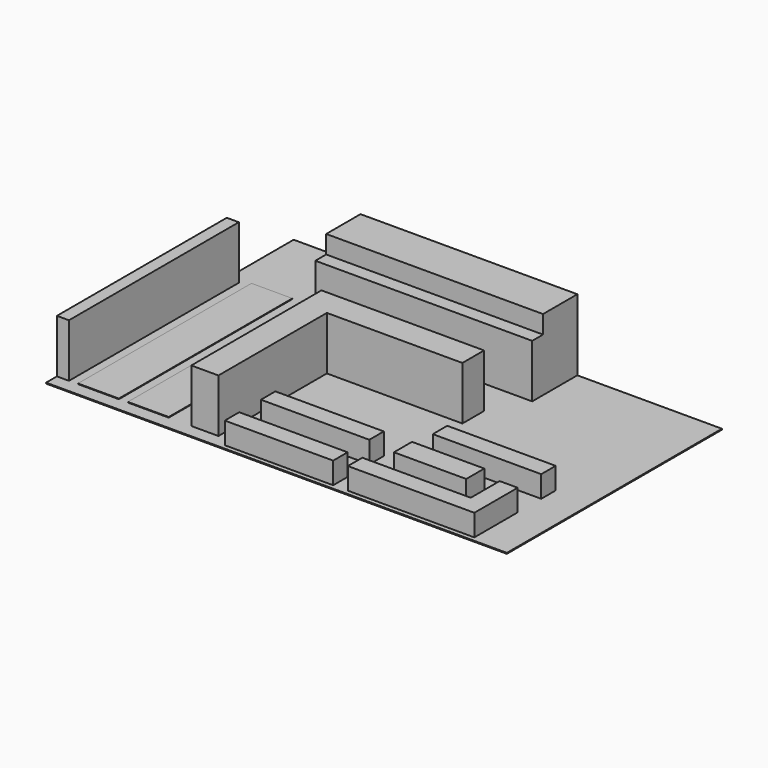
from build123d import *

# Parameters (mm, degrees)
F0_W     = 1377.95
F0_H     = 5486.4
F0_H_2   = 7315.2
F0_W_2   = 2438.4
F0_H_3   = 762
F0_W_3   = 3352.8
F0_H_4   = 1371.6
F0_W_4   = 914.4
F0_H_5   = 2438.4
F1_DEPTH = 30.48
F0_W_5   = 406.4
F0_H_6   = 7162.8
F0_W_6   = 7315.2
F0_H_7   = 457.2
F2_DEPTH = 1828.8
F0_W_7   = 1828.8
F0_H_8   = 609.6
F3_DEPTH = 762
F0_H_9   = 1447.8
F4_DEPTH = 2438.4
F6_DEPTH = 50.8
F0_W_8   = 457.2
F0_W_9   = 4572
F0_H_10  = 914.4
F7_DEPTH = 1828.8


# Not quite as in the source:
# - the program builds the solid bodies; features that only make, move or delete a surface that nothing else refers to are left out


with BuildPart() as f1:
    # F0 (on Top) → F1 (new body)
    with BuildSketch(Plane.XY):
        Polygon((3352.8, 9067.8), (0, 9067.8), (0, 7620), (406.4, 7620), (406.4, 457.2), (0, 457.2), (0, 0), (914.4, 0), (2438.4, 0), (5486.4, 0), (7010.4, 0), (13106.4, 0), (14630.4, 0), (14630.4, 2438.4), (15544.8, 2438.4), (15544.8, 3886.2), (10668, 3886.2), (10668, 7162.8), (3352.8, 7162.8), (3352.8, 7620), align=None)
        Polygon((5905.5, 1676.4), (5905.5, 2286), (7734.3, 2286), (9563.1, 2286), (9563.1, 1676.4), (9563.1, 762), (9563.1, 152.4), (7734.3, 152.4), (5905.5, 152.4), (5905.5, 762), align=None, mode=Mode.SUBTRACT)
        with Locations((3082.925, 3200.4)):
            Rectangle(F0_W, F0_H, mode=Mode.SUBTRACT)
        with Locations((1400.175, 4114.8)):
            Rectangle(F0_W, F0_H_2, mode=Mode.SUBTRACT)
        Polygon((4533.9, 457.2), (4533.9, 5943.6), (4991.1, 5943.6), (5448.3, 5943.6), (10020.3, 5943.6), (10020.3, 5029.2), (5448.3, 5029.2), (5448.3, 457.2), (4991.1, 457.2), align=None, mode=Mode.SUBTRACT)
        Polygon((12496.8, 3581.4), (14325.6, 3581.4), (14325.6, 2971.8), (14325.6, 1981.2), (14325.6, 152.4), (13716, 152.4), (11887.2, 152.4), (10058.4, 152.4), (9867.9, 152.4), (9867.9, 3581.4), (10668, 3581.4), align=None, mode=Mode.SUBTRACT)
        Polygon((14325.6, 1981.2), (14325.6, 2971.8), (12496.8, 2971.8), (10668, 2971.8), (10668, 3581.4), (9867.9, 3581.4), (9867.9, 152.4), (10058.4, 152.4), (10058.4, 762), (11887.2, 762), (13716, 762), (13716, 1981.2), align=None)
        with Locations((11734.8, 1905)):
            Rectangle(F0_W_2, F0_H_3, mode=Mode.SUBTRACT)
        Polygon((7734.3, 1676.4), (5905.5, 1676.4), (5905.5, 762), (7734.3, 762), (9563.1, 762), (9563.1, 1676.4), align=None)
        with Locations((1676.4, 9753.6)):
            Rectangle(F0_W_3, F0_H_4)
        Polygon((15544.8, 9067.8), (10668, 9067.8), (10668, 7620), (10668, 7162.8), (10668, 3886.2), (15544.8, 3886.2), align=None)
        with Locations((15087.6, 1219.2)):
            Rectangle(F0_W_4, F0_H_5)
    extrude(amount=F1_DEPTH)

    # F0 (on Top) → F2 (join)
    with BuildSketch(Plane.XY):
        with Locations((203.2, 4038.6)):
            Rectangle(F0_W_5, F0_H_6)
        with Locations((7010.4, 7391.4)):
            Rectangle(F0_W_6, F0_H_7)
    extrude(amount=F2_DEPTH)

    # F0 (on Top) → F3 (join)
    with BuildSketch(Plane.XY):
        with Locations((6819.9, 1981.2)):
            Rectangle(F0_W_7, F0_H_8)
        with Locations((8648.7, 1981.2)):
            Rectangle(F0_W_7, F0_H_8)
        with Locations((6819.9, 457.2)):
            Rectangle(F0_W_7, F0_H_8)
        with Locations((8648.7, 457.2)):
            Rectangle(F0_W_7, F0_H_8)
        with Locations((10972.8, 457.2)):
            Rectangle(F0_W_7, F0_H_8)
        with Locations((12801.6, 457.2)):
            Rectangle(F0_W_7, F0_H_8)
        Polygon((14325.6, 152.4), (14325.6, 1981.2), (13716, 1981.2), (13716, 762), (13716, 152.4), align=None)
        with Locations((11734.8, 1905)):
            Rectangle(F0_W_2, F0_H_3)
        with Locations((11582.4, 3276.6)):
            Rectangle(F0_W_7, F0_H_8)
        with Locations((13411.2, 3276.6)):
            Rectangle(F0_W_7, F0_H_8)
    extrude(amount=F3_DEPTH)

    # F0 (on Top) → F4 (join)
    with BuildSketch(Plane.XY):
        with Locations((7010.4, 8343.9)):
            Rectangle(F0_W_6, F0_H_9)
    extrude(amount=F4_DEPTH)

    # F0 (on Top) → F6 (join)
    with BuildSketch(Plane.XY):
        with Locations((1400.175, 4114.8)):
            Rectangle(F0_W, F0_H_2)
        with Locations((3082.925, 3200.4)):
            Rectangle(F0_W, F0_H)
    extrude(amount=F6_DEPTH)

    # F0 (on Top) → F7 (join)
    with BuildSketch(Plane.XY):
        with Locations((4762.5, 3200.4)):
            Rectangle(F0_W_8, F0_H)
        Polygon((5448.3, 5943.6), (4991.1, 5943.6), (4991.1, 457.2), (5448.3, 457.2), (5448.3, 5029.2), align=None)
        with Locations((7734.3, 5486.4)):
            Rectangle(F0_W_9, F0_H_10)
    extrude(amount=F7_DEPTH)


solid = f1.part
